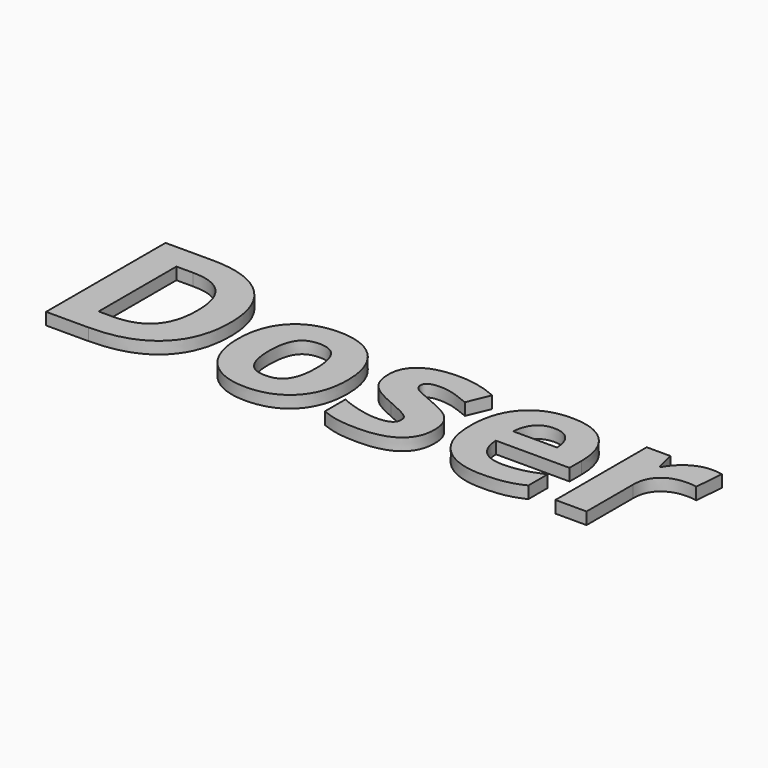
from build123d import *

# Parameters (mm, degrees)
F0_TEXT_SIZE = 34.7222222222
F1_DEPTH     = 2


# Not quite as in the source:
# - Text() gives the source's letters only with a copy of the font that has no kerning and outlines rounded to 1/6400 em; it was checked with that copy


with BuildPart() as f1:
    # F0 (on Top) → F1 (new body)
    with BuildSketch(Plane.XY):
        with Locations((-51.1338975694, -12.5)):
            Text('Doser', F0_TEXT_SIZE, font='Open Sans', font_style=FontStyle.BOLD, text_align=(TextAlign.LEFT, TextAlign.BOTTOM))
    extrude(amount=F1_DEPTH)


solid = f1.part
